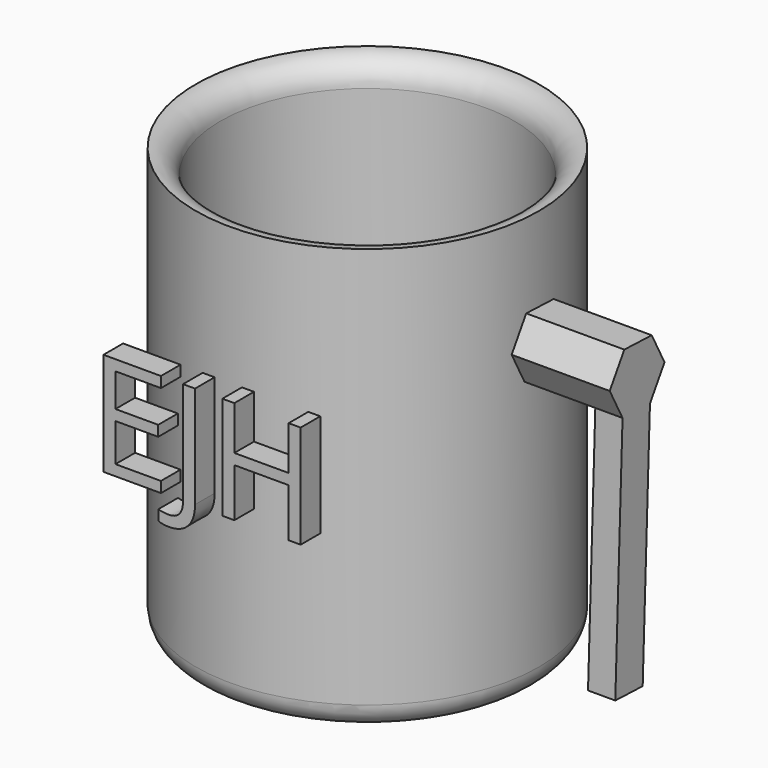
from build123d import *

# Parameters (mm, degrees)
F4_DEPTH     = 20
F5_W         = 5.5579461157
F5_H         = 6.9872754722
F6_DEPTH     = 50
F8_TEXT_SIZE = 29.4478527607
F9_DEPTH     = 5


# Not quite as in the source:
# - Text() gives the source's letters only with a copy of the font that has no kerning and outlines rounded to 1/6400 em; it was checked with that copy


with BuildPart() as f1:
    # F0 (on Front) → F1 (revolve)
    with BuildSketch(Plane.XZ):
        with BuildLine():
            ThreePointArc((35, 49.0476749837), (31.4644660941, 47.5832088897), (30, 44.0476749837))
            Line((30, 44.0476749837), (30, 37.1953517199))
            Line((30, 37.1953517199), (30, -25.7777617127))
            ThreePointArc((30, -25.7777617127), (28.5355339059, -29.3132956186), (25, -30.7777617127))
            Line((25, -30.7777617127), (0, -30.7777617127))
            Line((0, -30.7777617127), (0, -37.8046482801))
            Line((0, -37.8046482801), (30, -37.8046482801))
            ThreePointArc((30, -37.8046482801), (33.5355339059, -36.3401821861), (35, -32.8046482801))
            Line((35, -32.8046482801), (35, -30.7777617127))
            Line((35, -30.7777617127), (35, 32.1953517199))
            Line((35, 32.1953517199), (35, 49.0476749837))
        make_face()
    revolve(axis=Axis((0, 0, -2.7241725475), (0, 0, -1)))


with BuildPart() as f4:
    # F3 (on offset) → F4 (new body)
    with BuildSketch(Plane.YZ.offset(35)):
        Polygon((3.2670381711, 19.6466254734), (6.9824778707, 25.5641863192), (3.7154396996, 31.7406319082), (-3.2670381711, 31.9995166514), (-6.9824778707, 26.0819558056), (-3.7154396996, 19.9055102166), align=None)
    extrude(amount=F4_DEPTH)

    # F5 (on face) → F6 (join)
    with BuildSketch(Plane(origin=(0, 0.7319099483, 19.7406187565), x_dir=(1, 0, 0), z_dir=(0, -0.0370508855, -0.9993133802))):
        with Locations((52.2210269421, 0.9567676481)):
            Rectangle(F5_W, F5_H)
    extrude(amount=F6_DEPTH)


with BuildPart() as f9:
    # F8 (on offset) → F9 (new body)
    with BuildSketch(Plane.XZ.offset(35)):
        with Locations((-24.702730335, 0)):
            Text('EJH', F8_TEXT_SIZE, font='Open Sans', text_align=(TextAlign.LEFT, TextAlign.BOTTOM))
    extrude(amount=F9_DEPTH)


solid = Compound([f1.part, f4.part, f9.part])
